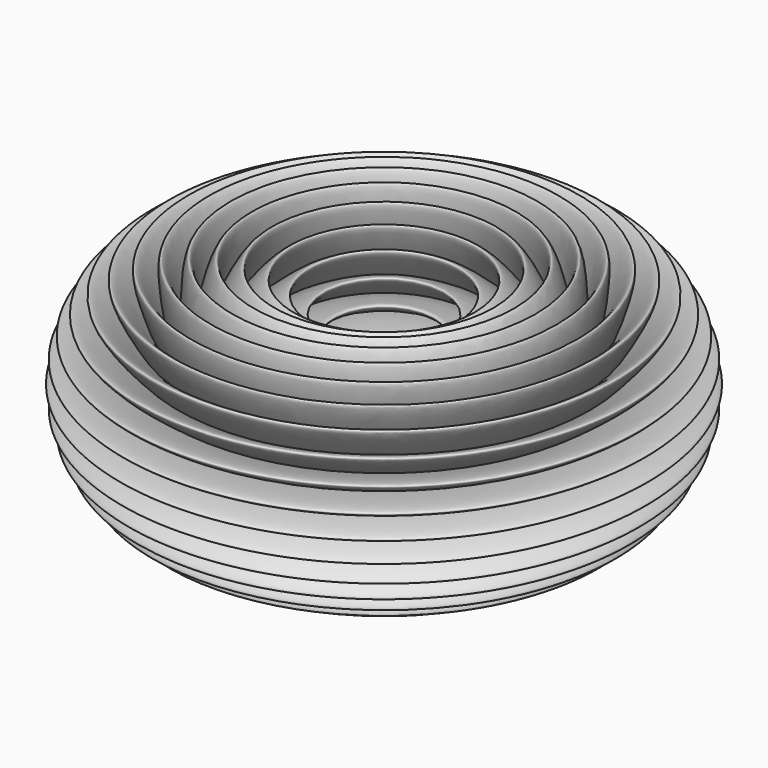
from build123d import *


with BuildPart() as f1:
    # F0 (on Front) → F1 (revolve)
    with BuildSketch(Plane.XZ):
        with BuildLine():
            add(Edge.make_bspline(
                [(306.7410461047, -30.2113560981), (430.4049725454, -21.4052719132), (586.5438764123, 0)],
                knots=[0.7817357195, 0.7817357195, 0.7817357195, 1.1221060483, 1.1221060483, 1.1221060483], degree=2, weights=[1, 0.9855534235, 1]))
            add(Edge.make_bspline(
                [(575.2736002958, -114.4290337258), (426.3108230752, -62.9738690757), (306.7410461047, -30.2113560981)],
                knots=[5.1610792589, 5.1610792589, 5.1610792589, 5.5014495877, 5.5014495877, 5.5014495877], degree=2, weights=[1, 0.9855534235, 1]))
            add(Edge.make_bspline(
                [(575.2736002958, -114.4290337259), (901.5747774696, -134.0658692103), (1253.6743252134, -123.4761436431)],
                knots=[1.1221060483, 1.1221060483, 1.1221060483, 1.8069156759, 1.8069156759, 1.8069156759], degree=2, weights=[1, 0.9419499659, 1]))
            add(Edge.make_bspline(
                [(1253.6743252134, -123.4761436431), (910.4062245206, -44.3986825322), (586.5438764123, 0)],
                knots=[4.4762696313, 4.4762696313, 4.4762696313, 5.1610792589, 5.1610792589, 5.1610792589], degree=2, weights=[1, 0.9419499659, 1]))
        make_face()
        with BuildLine():
            add(Edge.make_bspline(
                [(306.7410461047, 30.2113560981), (426.3108230753, 62.9738690757), (575.2736002958, 114.4290337258)],
                knots=[0.7817357195, 0.7817357195, 0.7817357195, 1.1221060483, 1.1221060483, 1.1221060483], degree=2, weights=[1, 0.9855534235, 1]))
            add(Edge.make_bspline(
                [(586.5438764123, 0), (430.4049725454, 21.4052719132), (306.7410461047, 30.2113560981)],
                knots=[5.1610792589, 5.1610792589, 5.1610792589, 5.5014495877, 5.5014495877, 5.5014495877], degree=2, weights=[1, 0.9855534235, 1]))
            add(Edge.make_bspline(
                [(586.5438764123, 0), (910.4062245206, 44.3986825322), (1253.6743252134, 123.4761436431)],
                knots=[1.1221060483, 1.1221060483, 1.1221060483, 1.8069156759, 1.8069156759, 1.8069156759], degree=2, weights=[1, 0.9419499659, 1]))
            add(Edge.make_bspline(
                [(1253.6743252134, 123.4761436431), (901.5747774696, 134.0658692103), (575.2736002958, 114.4290337259)],
                knots=[4.4762696313, 4.4762696313, 4.4762696313, 5.1610792589, 5.1610792589, 5.1610792589], degree=2, weights=[1, 0.9419499659, 1]))
        make_face()
        with BuildLine():
            add(Edge.make_bspline(
                [(294.9531597252, 89.4730628222), (405.8337877522, 144.9329595922), (541.8958823372, 224.4606238582)],
                knots=[0.7817357195, 0.7817357195, 0.7817357195, 1.1221060483, 1.1221060483, 1.1221060483], degree=2, weights=[1, 0.9855534235, 1]))
            add(Edge.make_bspline(
                [(575.2736002958, 114.4290337259), (417.9589002944, 104.9618203067), (294.9531597252, 89.4730628222)],
                knots=[5.1610792589, 5.1610792589, 5.1610792589, 5.5014495877, 5.5014495877, 5.5014495877], degree=2, weights=[1, 0.9855534235, 1]))
            add(Edge.make_bspline(
                [(575.2736002958, 114.4290337258), (884.251270925, 221.1570178041), (1205.4963239641, 365.6833119754)],
                knots=[1.1221060483, 1.1221060483, 1.1221060483, 1.8069156759, 1.8069156759, 1.8069156759], degree=2, weights=[1, 0.9419499659, 1]))
            add(Edge.make_bspline(
                [(1205.4963239641, 365.6833119754), (858.0963173294, 307.3783447841), (541.8958823372, 224.4606238582)],
                knots=[4.4762696313, 4.4762696313, 4.4762696313, 5.1610792589, 5.1610792589, 5.1610792589], degree=2, weights=[1, 0.9419499659, 1]))
        make_face()
        with BuildLine():
            add(Edge.make_bspline(
                [(575.2736002958, -114.4290337259), (901.5747774696, -134.0658692103), (1253.6743252134, -123.4761436431)],
                knots=[1.1221060483, 1.1221060483, 1.1221060483, 1.8069156759, 1.8069156759, 1.8069156759], degree=2, weights=[1, 0.9419499659, 1]))
            add(Edge.make_bspline(
                [(1205.4963239641, -365.6833119754), (884.251270925, -221.1570178041), (575.2736002958, -114.4290337258)],
                knots=[4.4762696313, 4.4762696313, 4.4762696313, 5.1610792589, 5.1610792589, 5.1610792589], degree=2, weights=[1, 0.9419499659, 1]))
            add(Edge.make_bspline(
                [(1205.4963239641, -365.6833119754), (1973.4335346691, -494.5680356943), (1992.9556897794, -396.4235343368), (2012.4778448897, -298.2790329793), (1253.6743252134, -123.4761436431)],
                knots=[1.8069156759, 1.8069156759, 1.8069156759, 3.1415926536, 3.1415926536, 4.4762696313, 4.4762696313, 4.4762696313], degree=2, weights=[1, 0.7854716489, 1, 0.7854716489, 1]))
        make_face()
        with BuildLine():
            add(Edge.make_bspline(
                [(1205.4963239641, -365.6833119754), (884.251270925, -221.1570178041), (575.2736002958, -114.4290337258)],
                knots=[4.4762696313, 4.4762696313, 4.4762696313, 5.1610792589, 5.1610792589, 5.1610792589], degree=2, weights=[1, 0.9419499659, 1]))
            add(Edge.make_bspline(
                [(294.9531597252, -89.4730628222), (417.9589002944, -104.9618203067), (575.2736002958, -114.4290337259)],
                knots=[0.7817357195, 0.7817357195, 0.7817357195, 1.1221060483, 1.1221060483, 1.1221060483], degree=2, weights=[1, 0.9855534235, 1]))
            add(Edge.make_bspline(
                [(541.8958823372, -224.4606238582), (405.8337877522, -144.9329595922), (294.9531597252, -89.4730628221)],
                knots=[5.1610792589, 5.1610792589, 5.1610792589, 5.5014495877, 5.5014495877, 5.5014495877], degree=2, weights=[1, 0.9855534235, 1]))
            add(Edge.make_bspline(
                [(541.8958823372, -224.4606238582), (858.0963173294, -307.3783447841), (1205.4963239641, -365.6833119754)],
                knots=[1.1221060483, 1.1221060483, 1.1221060483, 1.8069156759, 1.8069156759, 1.8069156759], degree=2, weights=[1, 0.9419499659, 1]))
        make_face()
        with BuildLine():
            add(Edge.make_bspline(
                [(586.5438764123, 0), (910.4062245206, 44.3986825322), (1253.6743252134, 123.4761436431)],
                knots=[1.1221060483, 1.1221060483, 1.1221060483, 1.8069156759, 1.8069156759, 1.8069156759], degree=2, weights=[1, 0.9419499659, 1]))
            add(Edge.make_bspline(
                [(1253.6743252134, -123.4761436431), (910.4062245206, -44.3986825322), (586.5438764123, 0)],
                knots=[4.4762696313, 4.4762696313, 4.4762696313, 5.1610792589, 5.1610792589, 5.1610792589], degree=2, weights=[1, 0.9419499659, 1]))
            add(Edge.make_bspline(
                [(1253.6743252134, -123.4761436431), (2032, -100.0672658109), (2032, 0), (2032, 100.0672658109), (1253.6743252134, 123.4761436431)],
                knots=[1.8069156759, 1.8069156759, 1.8069156759, 3.1415926536, 3.1415926536, 4.4762696313, 4.4762696313, 4.4762696313], degree=2, weights=[1, 0.7854716489, 1, 0.7854716489, 1]))
        make_face()
        with BuildLine():
            add(Edge.make_bspline(
                [(575.2736002958, 114.4290337258), (884.251270925, 221.1570178041), (1205.4963239641, 365.6833119754)],
                knots=[1.1221060483, 1.1221060483, 1.1221060483, 1.8069156759, 1.8069156759, 1.8069156759], degree=2, weights=[1, 0.9419499659, 1]))
            add(Edge.make_bspline(
                [(1253.6743252134, 123.4761436431), (901.5747774696, 134.0658692103), (575.2736002958, 114.4290337259)],
                knots=[4.4762696313, 4.4762696313, 4.4762696313, 5.1610792589, 5.1610792589, 5.1610792589], degree=2, weights=[1, 0.9419499659, 1]))
            add(Edge.make_bspline(
                [(1253.6743252134, 123.4761436431), (2012.4778448897, 298.2790329793), (1992.9556897794, 396.4235343368), (1973.4335346691, 494.5680356943), (1205.4963239641, 365.6833119754)],
                knots=[1.8069156759, 1.8069156759, 1.8069156759, 3.1415926536, 3.1415926536, 4.4762696313, 4.4762696313, 4.4762696313], degree=2, weights=[1, 0.7854716489, 1, 0.7854716489, 1]))
        make_face()
        with BuildLine():
            add(Edge.make_bspline(
                [(541.8958823372, 224.4606238582), (824.1150368816, 389.4164129081), (1110.991775035, 593.837475706)],
                knots=[1.1221060483, 1.1221060483, 1.1221060483, 1.8069156759, 1.8069156759, 1.8069156759], degree=2, weights=[1, 0.9419499659, 1]))
            add(Edge.make_bspline(
                [(1205.4963239641, 365.6833119754), (858.0963173294, 307.3783447841), (541.8958823372, 224.4606238582)],
                knots=[4.4762696313, 4.4762696313, 4.4762696313, 5.1610792589, 5.1610792589, 5.1610792589], degree=2, weights=[1, 0.9419499659, 1]))
            add(Edge.make_bspline(
                [(1205.4963239641, 365.6833119754), (1915.6172948108, 685.1626358088), (1877.3232100629, 777.6127345659), (1839.029125315, 870.0628333229), (1110.991775035, 593.837475706)],
                knots=[1.8069156759, 1.8069156759, 1.8069156759, 3.1415926536, 3.1415926536, 4.4762696313, 4.4762696313, 4.4762696313], degree=2, weights=[1, 0.7854716489, 1, 0.7854716489, 1]))
        make_face()
        with BuildLine():
            add(Edge.make_bspline(
                [(541.8958823372, 224.4606238582), (389.4509018993, 184.4847448091), (271.8303888292, 145.296369919)],
                knots=[5.1610792589, 5.1610792589, 5.1610792589, 5.5014495877, 5.5014495877, 5.5014495877], degree=2, weights=[1, 0.9855534235, 1]))
            add(Edge.make_bspline(
                [(541.8958823372, 224.4606238582), (824.1150368816, 389.4164129081), (1110.991775035, 593.837475706)],
                knots=[1.1221060483, 1.1221060483, 1.1221060483, 1.8069156759, 1.8069156759, 1.8069156759], degree=2, weights=[1, 0.9419499659, 1]))
            add(Edge.make_bspline(
                [(1110.991775035, 593.837475706), (781.6416969402, 468.8784429476), (487.6934095189, 325.8663180946)],
                knots=[4.4762696313, 4.4762696313, 4.4762696313, 5.1610792589, 5.1610792589, 5.1610792589], degree=2, weights=[1, 0.9419499659, 1]))
            add(Edge.make_bspline(
                [(271.8303888292, 145.296369919), (369.7607875601, 221.3223577509), (487.6934095189, 325.8663180946)],
                knots=[0.7817357195, 0.7817357195, 0.7817357195, 1.1221060483, 1.1221060483, 1.1221060483], degree=2, weights=[1, 0.9855534235, 1]))
        make_face()
        with BuildLine():
            add(Edge.make_bspline(
                [(1110.991775035, -593.8374757059), (1839.029125315, -870.0628333229), (1877.3232100629, -777.6127345659), (1915.6172948108, -685.1626358088), (1205.4963239641, -365.6833119754)],
                knots=[1.8069156759, 1.8069156759, 1.8069156759, 3.1415926536, 3.1415926536, 4.4762696313, 4.4762696313, 4.4762696313], degree=2, weights=[1, 0.7854716489, 1, 0.7854716489, 1]))
            add(Edge.make_bspline(
                [(541.8958823372, -224.4606238582), (858.0963173294, -307.3783447841), (1205.4963239641, -365.6833119754)],
                knots=[1.1221060483, 1.1221060483, 1.1221060483, 1.8069156759, 1.8069156759, 1.8069156759], degree=2, weights=[1, 0.9419499659, 1]))
            add(Edge.make_bspline(
                [(1110.991775035, -593.8374757059), (824.1150368816, -389.4164129081), (541.8958823372, -224.4606238582)],
                knots=[4.4762696313, 4.4762696313, 4.4762696313, 5.1610792589, 5.1610792589, 5.1610792589], degree=2, weights=[1, 0.9419499659, 1]))
        make_face()
        with BuildLine():
            add(Edge.make_bspline(
                [(1110.991775035, -593.8374757059), (824.1150368816, -389.4164129081), (541.8958823372, -224.4606238582)],
                knots=[4.4762696313, 4.4762696313, 4.4762696313, 5.1610792589, 5.1610792589, 5.1610792589], degree=2, weights=[1, 0.9419499659, 1]))
            add(Edge.make_bspline(
                [(271.8303888292, -145.296369919), (389.4509018993, -184.4847448091), (541.8958823372, -224.4606238582)],
                knots=[0.7817357195, 0.7817357195, 0.7817357195, 1.1221060483, 1.1221060483, 1.1221060483], degree=2, weights=[1, 0.9855534235, 1]))
            add(Edge.make_bspline(
                [(487.6934095189, -325.8663180946), (369.76078756, -221.3223577509), (271.8303888292, -145.296369919)],
                knots=[5.1610792589, 5.1610792589, 5.1610792589, 5.5014495877, 5.5014495877, 5.5014495877], degree=2, weights=[1, 0.9855534235, 1]))
            add(Edge.make_bspline(
                [(487.6934095189, -325.8663180946), (781.6416969401, -468.8784429476), (1110.991775035, -593.8374757059)],
                knots=[1.1221060483, 1.1221060483, 1.1221060483, 1.8069156759, 1.8069156759, 1.8069156759], degree=2, weights=[1, 0.9419499659, 1]))
        make_face()
        with BuildLine():
            add(Edge.make_bspline(
                [(1110.991775035, 593.837475706), (781.6416969402, 468.8784429476), (487.6934095189, 325.8663180946)],
                knots=[4.4762696313, 4.4762696313, 4.4762696313, 5.1610792589, 5.1610792589, 5.1610792589], degree=2, weights=[1, 0.9419499659, 1]))
            add(Edge.make_bspline(
                [(1110.991775035, 593.837475706), (1745.140646383, 1045.7158227879), (1689.5462521988, 1128.9187134958), (1633.9518580146, 1212.1216042038), (973.7924352426, 799.170798273)],
                knots=[1.8069156759, 1.8069156759, 1.8069156759, 3.1415926536, 3.1415926536, 4.4762696313, 4.4762696313, 4.4762696313], degree=2, weights=[1, 0.7854716489, 1, 0.7854716489, 1]))
            add(Edge.make_bspline(
                [(487.6934095189, 325.8663180946), (732.3085241398, 542.7107536512), (973.7924352426, 799.170798273)],
                knots=[1.1221060483, 1.1221060483, 1.1221060483, 1.8069156759, 1.8069156759, 1.8069156759], degree=2, weights=[1, 0.9419499659, 1]))
        make_face()
        with BuildLine():
            add(Edge.make_bspline(
                [(973.7924352426, -799.170798273), (1633.9518580146, -1212.1216042038), (1689.5462521988, -1128.9187134958), (1745.140646383, -1045.7158227879), (1110.991775035, -593.8374757059)],
                knots=[1.8069156759, 1.8069156759, 1.8069156759, 3.1415926536, 3.1415926536, 4.4762696313, 4.4762696313, 4.4762696313], degree=2, weights=[1, 0.7854716489, 1, 0.7854716489, 1]))
            add(Edge.make_bspline(
                [(487.6934095189, -325.8663180946), (781.6416969401, -468.8784429476), (1110.991775035, -593.8374757059)],
                knots=[1.1221060483, 1.1221060483, 1.1221060483, 1.8069156759, 1.8069156759, 1.8069156759], degree=2, weights=[1, 0.9419499659, 1]))
            add(Edge.make_bspline(
                [(973.7924352426, -799.170798273), (732.3085241398, -542.7107536512), (487.6934095189, -325.8663180946)],
                knots=[4.4762696313, 4.4762696313, 4.4762696313, 5.1610792589, 5.1610792589, 5.1610792589], degree=2, weights=[1, 0.9419499659, 1]))
        make_face()
        with BuildLine():
            add(Edge.make_bspline(
                [(487.6934095189, 325.8663180946), (345.9765237507, 256.9180240287), (238.2613285347, 195.5360190031)],
                knots=[5.1610792589, 5.1610792589, 5.1610792589, 5.5014495877, 5.5014495877, 5.5014495877], degree=2, weights=[1, 0.9855534235, 1]))
            add(Edge.make_bspline(
                [(487.6934095189, 325.8663180946), (732.3085241398, 542.7107536512), (973.7924352426, 799.170798273)],
                knots=[1.1221060483, 1.1221060483, 1.1221060483, 1.8069156759, 1.8069156759, 1.8069156759], degree=2, weights=[1, 0.9419499659, 1]))
            add(Edge.make_bspline(
                [(973.7924352426, 799.170798273), (675.1490244872, 612.3598054987), (414.7491524746, 414.7491524746)],
                knots=[4.4762696313, 4.4762696313, 4.4762696313, 5.1610792589, 5.1610792589, 5.1610792589], degree=2, weights=[1, 0.9419499659, 1]))
            add(Edge.make_bspline(
                [(238.2613285347, 195.5360190031), (319.4780876662, 289.2064618203), (414.7491524746, 414.7491524746)],
                knots=[0.7817357195, 0.7817357195, 0.7817357195, 1.1221060483, 1.1221060483, 1.1221060483], degree=2, weights=[1, 0.9855534235, 1]))
        make_face()
        with BuildLine():
            add(Edge.make_bspline(
                [(973.7924352426, 799.170798273), (675.1490244872, 612.3598054987), (414.7491524746, 414.7491524746)],
                knots=[4.4762696313, 4.4762696313, 4.4762696313, 5.1610792589, 5.1610792589, 5.1610792589], degree=2, weights=[1, 0.9419499659, 1]))
            add(Edge.make_bspline(
                [(973.7924352426, 799.170798273), (1507.5992216007, 1366.0827371414), (1436.8409793711, 1436.8409793711), (1366.0827371414, 1507.5992216007), (799.170798273, 973.7924352426)],
                knots=[1.8069156759, 1.8069156759, 1.8069156759, 3.1415926536, 3.1415926536, 4.4762696313, 4.4762696313, 4.4762696313], degree=2, weights=[1, 0.7854716489, 1, 0.7854716489, 1]))
            add(Edge.make_bspline(
                [(414.7491524746, 414.7491524746), (612.3598054987, 675.1490244872), (799.170798273, 973.7924352426)],
                knots=[1.1221060483, 1.1221060483, 1.1221060483, 1.8069156759, 1.8069156759, 1.8069156759], degree=2, weights=[1, 0.9419499659, 1]))
        make_face()
        with BuildLine():
            add(Edge.make_bspline(
                [(414.7491524746, -414.7491524746), (675.1490244872, -612.3598054987), (973.7924352426, -799.170798273)],
                knots=[1.1221060483, 1.1221060483, 1.1221060483, 1.8069156759, 1.8069156759, 1.8069156759], degree=2, weights=[1, 0.9419499659, 1]))
            add(Edge.make_bspline(
                [(973.7924352426, -799.170798273), (732.3085241398, -542.7107536512), (487.6934095189, -325.8663180946)],
                knots=[4.4762696313, 4.4762696313, 4.4762696313, 5.1610792589, 5.1610792589, 5.1610792589], degree=2, weights=[1, 0.9419499659, 1]))
            add(Edge.make_bspline(
                [(238.2613285347, -195.5360190031), (345.9765237507, -256.9180240287), (487.6934095189, -325.8663180946)],
                knots=[0.7817357195, 0.7817357195, 0.7817357195, 1.1221060483, 1.1221060483, 1.1221060483], degree=2, weights=[1, 0.9855534235, 1]))
            add(Edge.make_bspline(
                [(414.7491524746, -414.7491524746), (319.4780876662, -289.2064618203), (238.2613285347, -195.5360190031)],
                knots=[5.1610792589, 5.1610792589, 5.1610792589, 5.5014495877, 5.5014495877, 5.5014495877], degree=2, weights=[1, 0.9855534235, 1]))
        make_face()
        with BuildLine():
            add(Edge.make_bspline(
                [(799.170798273, -973.7924352426), (1366.0827371414, -1507.5992216008), (1436.8409793711, -1436.8409793711), (1507.5992216007, -1366.0827371414), (973.7924352426, -799.170798273)],
                knots=[1.8069156759, 1.8069156759, 1.8069156759, 3.1415926536, 3.1415926536, 4.4762696313, 4.4762696313, 4.4762696313], degree=2, weights=[1, 0.7854716489, 1, 0.7854716489, 1]))
            add(Edge.make_bspline(
                [(414.7491524746, -414.7491524746), (675.1490244872, -612.3598054987), (973.7924352426, -799.170798273)],
                knots=[1.1221060483, 1.1221060483, 1.1221060483, 1.8069156759, 1.8069156759, 1.8069156759], degree=2, weights=[1, 0.9419499659, 1]))
            add(Edge.make_bspline(
                [(799.170798273, -973.7924352426), (612.3598054987, -675.1490244873), (414.7491524746, -414.7491524746)],
                knots=[4.4762696313, 4.4762696313, 4.4762696313, 5.1610792589, 5.1610792589, 5.1610792589], degree=2, weights=[1, 0.9419499659, 1]))
        make_face()
        with BuildLine():
            add(Edge.make_bspline(
                [(414.7491524746, 414.7491524746), (289.2064618203, 319.4780876662), (195.5360190031, 238.2613285347)],
                knots=[5.1610792589, 5.1610792589, 5.1610792589, 5.5014495877, 5.5014495877, 5.5014495877], degree=2, weights=[1, 0.9855534235, 1]))
            add(Edge.make_bspline(
                [(414.7491524746, 414.7491524746), (612.3598054987, 675.1490244872), (799.170798273, 973.7924352426)],
                knots=[1.1221060483, 1.1221060483, 1.1221060483, 1.8069156759, 1.8069156759, 1.8069156759], degree=2, weights=[1, 0.9419499659, 1]))
            add(Edge.make_bspline(
                [(799.170798273, 973.7924352426), (542.7107536512, 732.3085241398), (325.8663180946, 487.6934095189)],
                knots=[4.4762696313, 4.4762696313, 4.4762696313, 5.1610792589, 5.1610792589, 5.1610792589], degree=2, weights=[1, 0.9419499659, 1]))
            add(Edge.make_bspline(
                [(195.5360190031, 238.2613285347), (256.9180240287, 345.9765237507), (325.8663180946, 487.6934095189)],
                knots=[0.7817357195, 0.7817357195, 0.7817357195, 1.1221060483, 1.1221060483, 1.1221060483], degree=2, weights=[1, 0.9855534235, 1]))
        make_face()
        with BuildLine():
            add(Edge.make_bspline(
                [(799.170798273, 973.7924352426), (542.7107536512, 732.3085241398), (325.8663180946, 487.6934095189)],
                knots=[4.4762696313, 4.4762696313, 4.4762696313, 5.1610792589, 5.1610792589, 5.1610792589], degree=2, weights=[1, 0.9419499659, 1]))
            add(Edge.make_bspline(
                [(799.170798273, 973.7924352426), (1212.1216042038, 1633.9518580145), (1128.9187134958, 1689.5462521988), (1045.7158227879, 1745.140646383), (593.837475706, 1110.991775035)],
                knots=[1.8069156759, 1.8069156759, 1.8069156759, 3.1415926536, 3.1415926536, 4.4762696313, 4.4762696313, 4.4762696313], degree=2, weights=[1, 0.7854716489, 1, 0.7854716489, 1]))
            add(Edge.make_bspline(
                [(325.8663180946, 487.6934095189), (468.8784429476, 781.6416969402), (593.837475706, 1110.9917750351)],
                knots=[1.1221060483, 1.1221060483, 1.1221060483, 1.8069156759, 1.8069156759, 1.8069156759], degree=2, weights=[1, 0.9419499659, 1]))
        make_face()
        with BuildLine():
            add(Edge.make_bspline(
                [(325.8663180946, -487.6934095189), (542.7107536512, -732.3085241398), (799.170798273, -973.7924352426)],
                knots=[1.1221060483, 1.1221060483, 1.1221060483, 1.8069156759, 1.8069156759, 1.8069156759], degree=2, weights=[1, 0.9419499659, 1]))
            add(Edge.make_bspline(
                [(799.170798273, -973.7924352426), (612.3598054987, -675.1490244873), (414.7491524746, -414.7491524746)],
                knots=[4.4762696313, 4.4762696313, 4.4762696313, 5.1610792589, 5.1610792589, 5.1610792589], degree=2, weights=[1, 0.9419499659, 1]))
            add(Edge.make_bspline(
                [(195.5360190031, -238.2613285347), (289.2064618203, -319.4780876662), (414.7491524746, -414.7491524746)],
                knots=[0.7817357195, 0.7817357195, 0.7817357195, 1.1221060483, 1.1221060483, 1.1221060483], degree=2, weights=[1, 0.9855534235, 1]))
            add(Edge.make_bspline(
                [(325.8663180946, -487.6934095189), (256.9180240287, -345.9765237507), (195.5360190031, -238.2613285347)],
                knots=[5.1610792589, 5.1610792589, 5.1610792589, 5.5014495877, 5.5014495877, 5.5014495877], degree=2, weights=[1, 0.9855534235, 1]))
        make_face()
        with BuildLine():
            add(Edge.make_bspline(
                [(593.8374757059, -1110.991775035), (1045.7158227879, -1745.140646383), (1128.9187134958, -1689.5462521988), (1212.1216042038, -1633.9518580146), (799.170798273, -973.7924352426)],
                knots=[1.8069156759, 1.8069156759, 1.8069156759, 3.1415926536, 3.1415926536, 4.4762696313, 4.4762696313, 4.4762696313], degree=2, weights=[1, 0.7854716489, 1, 0.7854716489, 1]))
            add(Edge.make_bspline(
                [(325.8663180946, -487.6934095189), (542.7107536512, -732.3085241398), (799.170798273, -973.7924352426)],
                knots=[1.1221060483, 1.1221060483, 1.1221060483, 1.8069156759, 1.8069156759, 1.8069156759], degree=2, weights=[1, 0.9419499659, 1]))
            add(Edge.make_bspline(
                [(593.8374757059, -1110.991775035), (468.8784429476, -781.6416969402), (325.8663180946, -487.6934095189)],
                knots=[4.4762696313, 4.4762696313, 4.4762696313, 5.1610792589, 5.1610792589, 5.1610792589], degree=2, weights=[1, 0.9419499659, 1]))
        make_face()
        with BuildLine():
            add(Edge.make_bspline(
                [(593.837475706, 1110.991775035), (389.4164129081, 824.1150368816), (224.4606238582, 541.8958823372)],
                knots=[4.4762696313, 4.4762696313, 4.4762696313, 5.1610792589, 5.1610792589, 5.1610792589], degree=2, weights=[1, 0.9419499659, 1]))
            add(Edge.make_bspline(
                [(593.837475706, 1110.9917750351), (870.0628333229, 1839.0291253151), (777.6127345659, 1877.3232100629), (685.1626358088, 1915.6172948108), (365.6833119754, 1205.4963239641)],
                knots=[1.8069156759, 1.8069156759, 1.8069156759, 3.1415926536, 3.1415926536, 4.4762696313, 4.4762696313, 4.4762696313], degree=2, weights=[1, 0.7854716489, 1, 0.7854716489, 1]))
            add(Edge.make_bspline(
                [(224.4606238582, 541.8958823372), (307.3783447841, 858.0963173294), (365.6833119754, 1205.4963239641)],
                knots=[1.1221060483, 1.1221060483, 1.1221060483, 1.8069156759, 1.8069156759, 1.8069156759], degree=2, weights=[1, 0.9419499659, 1]))
        make_face()
        with BuildLine():
            add(Edge.make_bspline(
                [(325.8663180946, 487.6934095189), (468.8784429476, 781.6416969402), (593.837475706, 1110.9917750351)],
                knots=[1.1221060483, 1.1221060483, 1.1221060483, 1.8069156759, 1.8069156759, 1.8069156759], degree=2, weights=[1, 0.9419499659, 1]))
            add(Edge.make_bspline(
                [(593.837475706, 1110.991775035), (389.4164129081, 824.1150368816), (224.4606238582, 541.8958823372)],
                knots=[4.4762696313, 4.4762696313, 4.4762696313, 5.1610792589, 5.1610792589, 5.1610792589], degree=2, weights=[1, 0.9419499659, 1]))
            add(Edge.make_bspline(
                [(145.296369919, 271.8303888292), (184.4847448091, 389.4509018993), (224.4606238582, 541.8958823372)],
                knots=[0.7817357195, 0.7817357195, 0.7817357195, 1.1221060483, 1.1221060483, 1.1221060483], degree=2, weights=[1, 0.9855534235, 1]))
            add(Edge.make_bspline(
                [(325.8663180946, 487.6934095189), (221.3223577509, 369.7607875601), (145.296369919, 271.8303888292)],
                knots=[5.1610792589, 5.1610792589, 5.1610792589, 5.5014495877, 5.5014495877, 5.5014495877], degree=2, weights=[1, 0.9855534235, 1]))
        make_face()
        with BuildLine():
            add(Edge.make_bspline(
                [(365.6833119753, -1205.4963239641), (685.1626358088, -1915.6172948108), (777.6127345659, -1877.3232100629), (870.0628333229, -1839.029125315), (593.8374757059, -1110.991775035)],
                knots=[1.8069156759, 1.8069156759, 1.8069156759, 3.1415926536, 3.1415926536, 4.4762696313, 4.4762696313, 4.4762696313], degree=2, weights=[1, 0.7854716489, 1, 0.7854716489, 1]))
            add(Edge.make_bspline(
                [(224.4606238582, -541.8958823372), (389.4164129081, -824.1150368816), (593.8374757059, -1110.991775035)],
                knots=[1.1221060483, 1.1221060483, 1.1221060483, 1.8069156759, 1.8069156759, 1.8069156759], degree=2, weights=[1, 0.9419499659, 1]))
            add(Edge.make_bspline(
                [(365.6833119753, -1205.4963239641), (307.3783447841, -858.0963173294), (224.4606238582, -541.8958823372)],
                knots=[4.4762696313, 4.4762696313, 4.4762696313, 5.1610792589, 5.1610792589, 5.1610792589], degree=2, weights=[1, 0.9419499659, 1]))
        make_face()
        with BuildLine():
            add(Edge.make_bspline(
                [(224.4606238582, -541.8958823372), (389.4164129081, -824.1150368816), (593.8374757059, -1110.991775035)],
                knots=[1.1221060483, 1.1221060483, 1.1221060483, 1.8069156759, 1.8069156759, 1.8069156759], degree=2, weights=[1, 0.9419499659, 1]))
            add(Edge.make_bspline(
                [(593.8374757059, -1110.991775035), (468.8784429476, -781.6416969402), (325.8663180946, -487.6934095189)],
                knots=[4.4762696313, 4.4762696313, 4.4762696313, 5.1610792589, 5.1610792589, 5.1610792589], degree=2, weights=[1, 0.9419499659, 1]))
            add(Edge.make_bspline(
                [(145.296369919, -271.8303888292), (221.3223577509, -369.7607875601), (325.8663180946, -487.6934095189)],
                knots=[0.7817357195, 0.7817357195, 0.7817357195, 1.1221060483, 1.1221060483, 1.1221060483], degree=2, weights=[1, 0.9855534235, 1]))
            add(Edge.make_bspline(
                [(224.4606238582, -541.8958823372), (184.4847448091, -389.4509018993), (145.296369919, -271.8303888292)],
                knots=[5.1610792589, 5.1610792589, 5.1610792589, 5.5014495877, 5.5014495877, 5.5014495877], degree=2, weights=[1, 0.9855534235, 1]))
        make_face()
        with BuildLine():
            add(Edge.make_bspline(
                [(365.6833119754, 1205.4963239641), (221.1570178041, 884.251270925), (114.4290337258, 575.2736002958)],
                knots=[4.4762696313, 4.4762696313, 4.4762696313, 5.1610792589, 5.1610792589, 5.1610792589], degree=2, weights=[1, 0.9419499659, 1]))
            add(Edge.make_bspline(
                [(365.6833119754, 1205.4963239641), (494.5680356943, 1973.4335346691), (396.4235343368, 1992.9556897794), (298.2790329793, 2012.4778448897), (123.4761436431, 1253.6743252134)],
                knots=[1.8069156759, 1.8069156759, 1.8069156759, 3.1415926536, 3.1415926536, 4.4762696313, 4.4762696313, 4.4762696313], degree=2, weights=[1, 0.7854716489, 1, 0.7854716489, 1]))
            add(Edge.make_bspline(
                [(114.4290337259, 575.2736002958), (134.0658692103, 901.5747774696), (123.4761436431, 1253.6743252134)],
                knots=[1.1221060483, 1.1221060483, 1.1221060483, 1.8069156759, 1.8069156759, 1.8069156759], degree=2, weights=[1, 0.9419499659, 1]))
        make_face()
        with BuildLine():
            add(Edge.make_bspline(
                [(224.4606238582, 541.8958823372), (307.3783447841, 858.0963173294), (365.6833119754, 1205.4963239641)],
                knots=[1.1221060483, 1.1221060483, 1.1221060483, 1.8069156759, 1.8069156759, 1.8069156759], degree=2, weights=[1, 0.9419499659, 1]))
            add(Edge.make_bspline(
                [(365.6833119754, 1205.4963239641), (221.1570178041, 884.251270925), (114.4290337258, 575.2736002958)],
                knots=[4.4762696313, 4.4762696313, 4.4762696313, 5.1610792589, 5.1610792589, 5.1610792589], degree=2, weights=[1, 0.9419499659, 1]))
            add(Edge.make_bspline(
                [(89.4730628222, 294.9531597252), (104.9618203067, 417.9589002944), (114.4290337259, 575.2736002958)],
                knots=[0.7817357195, 0.7817357195, 0.7817357195, 1.1221060483, 1.1221060483, 1.1221060483], degree=2, weights=[1, 0.9855534235, 1]))
            add(Edge.make_bspline(
                [(224.4606238582, 541.8958823372), (144.9329595922, 405.8337877522), (89.4730628222, 294.9531597252)],
                knots=[5.1610792589, 5.1610792589, 5.1610792589, 5.5014495877, 5.5014495877, 5.5014495877], degree=2, weights=[1, 0.9855534235, 1]))
        make_face()
        with BuildLine():
            add(Edge.make_bspline(
                [(365.6833119753, -1205.4963239641), (307.3783447841, -858.0963173294), (224.4606238582, -541.8958823372)],
                knots=[4.4762696313, 4.4762696313, 4.4762696313, 5.1610792589, 5.1610792589, 5.1610792589], degree=2, weights=[1, 0.9419499659, 1]))
            add(Edge.make_bspline(
                [(89.4730628221, -294.9531597252), (144.9329595922, -405.8337877522), (224.4606238582, -541.8958823372)],
                knots=[0.7817357195, 0.7817357195, 0.7817357195, 1.1221060483, 1.1221060483, 1.1221060483], degree=2, weights=[1, 0.9855534235, 1]))
            add(Edge.make_bspline(
                [(114.4290337259, -575.2736002958), (104.9618203067, -417.9589002944), (89.4730628222, -294.9531597252)],
                knots=[5.1610792589, 5.1610792589, 5.1610792589, 5.5014495877, 5.5014495877, 5.5014495877], degree=2, weights=[1, 0.9855534235, 1]))
            add(Edge.make_bspline(
                [(114.4290337258, -575.2736002958), (221.1570178041, -884.251270925), (365.6833119753, -1205.4963239641)],
                knots=[1.1221060483, 1.1221060483, 1.1221060483, 1.8069156759, 1.8069156759, 1.8069156759], degree=2, weights=[1, 0.9419499659, 1]))
        make_face()
        with BuildLine():
            add(Edge.make_bspline(
                [(123.4761436431, -1253.6743252134), (298.2790329793, -2012.4778448897), (396.4235343368, -1992.9556897794), (494.5680356943, -1973.433534669), (365.6833119753, -1205.4963239641)],
                knots=[1.8069156759, 1.8069156759, 1.8069156759, 3.1415926536, 3.1415926536, 4.4762696313, 4.4762696313, 4.4762696313], degree=2, weights=[1, 0.7854716489, 1, 0.7854716489, 1]))
            add(Edge.make_bspline(
                [(114.4290337258, -575.2736002958), (221.1570178041, -884.251270925), (365.6833119753, -1205.4963239641)],
                knots=[1.1221060483, 1.1221060483, 1.1221060483, 1.8069156759, 1.8069156759, 1.8069156759], degree=2, weights=[1, 0.9419499659, 1]))
            add(Edge.make_bspline(
                [(123.4761436431, -1253.6743252134), (134.0658692103, -901.5747774696), (114.4290337259, -575.2736002958)],
                knots=[4.4762696313, 4.4762696313, 4.4762696313, 5.1610792589, 5.1610792589, 5.1610792589], degree=2, weights=[1, 0.9419499659, 1]))
        make_face()
        with BuildLine():
            add(Edge.make_bspline(
                [(123.4761436431, 1253.6743252134), (44.3986825322, 910.4062245206), (0, 586.5438764123)],
                knots=[4.4762696313, 4.4762696313, 4.4762696313, 5.1610792589, 5.1610792589, 5.1610792589], degree=2, weights=[1, 0.9419499659, 1]))
            add(Edge.make_bspline(
                [(123.4761436431, 1253.6743252134), (100.0672658109, 2032), (0, 2032), (-100.0672658109, 2032), (-123.4761436431, 1253.6743252133)],
                knots=[1.8069156759, 1.8069156759, 1.8069156759, 3.1415926536, 3.1415926536, 4.4762696313, 4.4762696313, 4.4762696313], degree=2, weights=[1, 0.7854716489, 1, 0.7854716489, 1]))
            add(Edge.make_bspline(
                [(0, 586.5438764123), (-44.3986825322, 910.4062245206), (-123.4761436431, 1253.6743252134)],
                knots=[1.1221060483, 1.1221060483, 1.1221060483, 1.8069156759, 1.8069156759, 1.8069156759], degree=2, weights=[1, 0.9419499659, 1]))
        make_face()
        with BuildLine():
            add(Edge.make_bspline(
                [(114.4290337259, 575.2736002958), (134.0658692103, 901.5747774696), (123.4761436431, 1253.6743252134)],
                knots=[1.1221060483, 1.1221060483, 1.1221060483, 1.8069156759, 1.8069156759, 1.8069156759], degree=2, weights=[1, 0.9419499659, 1]))
            add(Edge.make_bspline(
                [(123.4761436431, 1253.6743252134), (44.3986825322, 910.4062245206), (0, 586.5438764123)],
                knots=[4.4762696313, 4.4762696313, 4.4762696313, 5.1610792589, 5.1610792589, 5.1610792589], degree=2, weights=[1, 0.9419499659, 1]))
            add(Edge.make_bspline(
                [(30.2113560981, 306.7410461047), (21.4052719132, 430.4049725454), (0, 586.5438764123)],
                knots=[0.7817357195, 0.7817357195, 0.7817357195, 1.1221060483, 1.1221060483, 1.1221060483], degree=2, weights=[1, 0.9855534235, 1]))
            add(Edge.make_bspline(
                [(114.4290337258, 575.2736002958), (62.9738690757, 426.3108230752), (30.2113560981, 306.7410461047)],
                knots=[5.1610792589, 5.1610792589, 5.1610792589, 5.5014495877, 5.5014495877, 5.5014495877], degree=2, weights=[1, 0.9855534235, 1]))
        make_face()
        with BuildLine():
            add(Edge.make_bspline(
                [(123.4761436431, -1253.6743252134), (134.0658692103, -901.5747774696), (114.4290337259, -575.2736002958)],
                knots=[4.4762696313, 4.4762696313, 4.4762696313, 5.1610792589, 5.1610792589, 5.1610792589], degree=2, weights=[1, 0.9419499659, 1]))
            add(Edge.make_bspline(
                [(30.2113560981, -306.7410461047), (62.9738690757, -426.3108230752), (114.4290337258, -575.2736002958)],
                knots=[0.7817357195, 0.7817357195, 0.7817357195, 1.1221060483, 1.1221060483, 1.1221060483], degree=2, weights=[1, 0.9855534235, 1]))
            add(Edge.make_bspline(
                [(0, -586.5438764123), (21.4052719132, -430.4049725454), (30.2113560981, -306.7410461047)],
                knots=[5.1610792589, 5.1610792589, 5.1610792589, 5.5014495877, 5.5014495877, 5.5014495877], degree=2, weights=[1, 0.9855534235, 1]))
            add(Edge.make_bspline(
                [(0, -586.5438764123), (44.3986825322, -910.4062245206), (123.4761436431, -1253.6743252134)],
                knots=[1.1221060483, 1.1221060483, 1.1221060483, 1.8069156759, 1.8069156759, 1.8069156759], degree=2, weights=[1, 0.9419499659, 1]))
        make_face()
        with BuildLine():
            add(Edge.make_bspline(
                [(-123.4761436431, -1253.6743252134), (-100.0672658109, -2032), (0, -2032), (100.0672658109, -2032), (123.4761436431, -1253.6743252134)],
                knots=[1.8069156759, 1.8069156759, 1.8069156759, 3.1415926536, 3.1415926536, 4.4762696313, 4.4762696313, 4.4762696313], degree=2, weights=[1, 0.7854716489, 1, 0.7854716489, 1]))
            add(Edge.make_bspline(
                [(0, -586.5438764123), (44.3986825322, -910.4062245206), (123.4761436431, -1253.6743252134)],
                knots=[1.1221060483, 1.1221060483, 1.1221060483, 1.8069156759, 1.8069156759, 1.8069156759], degree=2, weights=[1, 0.9419499659, 1]))
            add(Edge.make_bspline(
                [(-123.4761436431, -1253.6743252134), (-44.3986825322, -910.4062245206), (0, -586.5438764123)],
                knots=[4.4762696313, 4.4762696313, 4.4762696313, 5.1610792589, 5.1610792589, 5.1610792589], degree=2, weights=[1, 0.9419499659, 1]))
        make_face()
        with BuildLine():
            add(Edge.make_bspline(
                [(0, 586.5438764123), (-44.3986825322, 910.4062245206), (-123.4761436431, 1253.6743252134)],
                knots=[1.1221060483, 1.1221060483, 1.1221060483, 1.8069156759, 1.8069156759, 1.8069156759], degree=2, weights=[1, 0.9419499659, 1]))
            add(Edge.make_bspline(
                [(-123.4761436431, 1253.6743252133), (-134.0658692103, 901.5747774696), (-114.4290337259, 575.2736002958)],
                knots=[4.4762696313, 4.4762696313, 4.4762696313, 5.1610792589, 5.1610792589, 5.1610792589], degree=2, weights=[1, 0.9419499659, 1]))
            add(Edge.make_bspline(
                [(-30.2113560981, 306.7410461047), (-62.9738690757, 426.3108230752), (-114.4290337258, 575.2736002958)],
                knots=[0.7817357195, 0.7817357195, 0.7817357195, 1.1221060483, 1.1221060483, 1.1221060483], degree=2, weights=[1, 0.9855534235, 1]))
            add(Edge.make_bspline(
                [(0, 586.5438764123), (-21.4052719132, 430.4049725454), (-30.2113560981, 306.7410461047)],
                knots=[5.1610792589, 5.1610792589, 5.1610792589, 5.5014495877, 5.5014495877, 5.5014495877], degree=2, weights=[1, 0.9855534235, 1]))
        make_face()
        with BuildLine():
            add(Edge.make_bspline(
                [(-123.4761436431, 1253.6743252133), (-134.0658692103, 901.5747774696), (-114.4290337259, 575.2736002958)],
                knots=[4.4762696313, 4.4762696313, 4.4762696313, 5.1610792589, 5.1610792589, 5.1610792589], degree=2, weights=[1, 0.9419499659, 1]))
            add(Edge.make_bspline(
                [(-123.4761436431, 1253.6743252134), (-298.2790329793, 2012.4778448897), (-396.4235343368, 1992.9556897794), (-494.5680356943, 1973.4335346691), (-365.6833119754, 1205.4963239641)],
                knots=[1.8069156759, 1.8069156759, 1.8069156759, 3.1415926536, 3.1415926536, 4.4762696313, 4.4762696313, 4.4762696313], degree=2, weights=[1, 0.7854716489, 1, 0.7854716489, 1]))
            add(Edge.make_bspline(
                [(-114.4290337258, 575.2736002958), (-221.1570178041, 884.251270925), (-365.6833119754, 1205.4963239641)],
                knots=[1.1221060483, 1.1221060483, 1.1221060483, 1.8069156759, 1.8069156759, 1.8069156759], degree=2, weights=[1, 0.9419499659, 1]))
        make_face()
        with BuildLine():
            add(Edge.make_bspline(
                [(-123.4761436431, -1253.6743252134), (-44.3986825322, -910.4062245206), (0, -586.5438764123)],
                knots=[4.4762696313, 4.4762696313, 4.4762696313, 5.1610792589, 5.1610792589, 5.1610792589], degree=2, weights=[1, 0.9419499659, 1]))
            add(Edge.make_bspline(
                [(-30.2113560981, -306.7410461047), (-21.4052719132, -430.4049725454), (0, -586.5438764123)],
                knots=[0.7817357195, 0.7817357195, 0.7817357195, 1.1221060483, 1.1221060483, 1.1221060483], degree=2, weights=[1, 0.9855534235, 1]))
            add(Edge.make_bspline(
                [(-114.4290337258, -575.2736002958), (-62.9738690757, -426.3108230753), (-30.2113560981, -306.7410461047)],
                knots=[5.1610792589, 5.1610792589, 5.1610792589, 5.5014495877, 5.5014495877, 5.5014495877], degree=2, weights=[1, 0.9855534235, 1]))
            add(Edge.make_bspline(
                [(-114.4290337259, -575.2736002958), (-134.0658692103, -901.5747774696), (-123.4761436431, -1253.6743252134)],
                knots=[1.1221060483, 1.1221060483, 1.1221060483, 1.8069156759, 1.8069156759, 1.8069156759], degree=2, weights=[1, 0.9419499659, 1]))
        make_face()
        with BuildLine():
            add(Edge.make_bspline(
                [(-365.6833119754, -1205.4963239641), (-494.5680356943, -1973.433534669), (-396.4235343368, -1992.9556897794), (-298.2790329793, -2012.4778448897), (-123.4761436431, -1253.6743252134)],
                knots=[1.8069156759, 1.8069156759, 1.8069156759, 3.1415926536, 3.1415926536, 4.4762696313, 4.4762696313, 4.4762696313], degree=2, weights=[1, 0.7854716489, 1, 0.7854716489, 1]))
            add(Edge.make_bspline(
                [(-114.4290337259, -575.2736002958), (-134.0658692103, -901.5747774696), (-123.4761436431, -1253.6743252134)],
                knots=[1.1221060483, 1.1221060483, 1.1221060483, 1.8069156759, 1.8069156759, 1.8069156759], degree=2, weights=[1, 0.9419499659, 1]))
            add(Edge.make_bspline(
                [(-365.6833119754, -1205.4963239641), (-221.1570178041, -884.251270925), (-114.4290337258, -575.2736002958)],
                knots=[4.4762696313, 4.4762696313, 4.4762696313, 5.1610792589, 5.1610792589, 5.1610792589], degree=2, weights=[1, 0.9419499659, 1]))
        make_face()
        with BuildLine():
            add(Edge.make_bspline(
                [(-114.4290337259, 575.2736002958), (-104.9618203067, 417.9589002944), (-89.4730628222, 294.9531597252)],
                knots=[5.1610792589, 5.1610792589, 5.1610792589, 5.5014495877, 5.5014495877, 5.5014495877], degree=2, weights=[1, 0.9855534235, 1]))
            add(Edge.make_bspline(
                [(-114.4290337258, 575.2736002958), (-221.1570178041, 884.251270925), (-365.6833119754, 1205.4963239641)],
                knots=[1.1221060483, 1.1221060483, 1.1221060483, 1.8069156759, 1.8069156759, 1.8069156759], degree=2, weights=[1, 0.9419499659, 1]))
            add(Edge.make_bspline(
                [(-365.6833119754, 1205.4963239641), (-307.3783447841, 858.0963173294), (-224.4606238582, 541.8958823372)],
                knots=[4.4762696313, 4.4762696313, 4.4762696313, 5.1610792589, 5.1610792589, 5.1610792589], degree=2, weights=[1, 0.9419499659, 1]))
            add(Edge.make_bspline(
                [(-89.4730628221, 294.9531597252), (-144.9329595922, 405.8337877522), (-224.4606238582, 541.8958823372)],
                knots=[0.7817357195, 0.7817357195, 0.7817357195, 1.1221060483, 1.1221060483, 1.1221060483], degree=2, weights=[1, 0.9855534235, 1]))
        make_face()
        with BuildLine():
            add(Edge.make_bspline(
                [(-365.6833119754, 1205.4963239641), (-307.3783447841, 858.0963173294), (-224.4606238582, 541.8958823372)],
                knots=[4.4762696313, 4.4762696313, 4.4762696313, 5.1610792589, 5.1610792589, 5.1610792589], degree=2, weights=[1, 0.9419499659, 1]))
            add(Edge.make_bspline(
                [(-365.6833119754, 1205.4963239641), (-685.1626358088, 1915.6172948108), (-777.6127345659, 1877.3232100629), (-870.0628333229, 1839.029125315), (-593.8374757059, 1110.991775035)],
                knots=[1.8069156759, 1.8069156759, 1.8069156759, 3.1415926536, 3.1415926536, 4.4762696313, 4.4762696313, 4.4762696313], degree=2, weights=[1, 0.7854716489, 1, 0.7854716489, 1]))
            add(Edge.make_bspline(
                [(-224.4606238582, 541.8958823372), (-389.4164129081, 824.1150368816), (-593.8374757059, 1110.991775035)],
                knots=[1.1221060483, 1.1221060483, 1.1221060483, 1.8069156759, 1.8069156759, 1.8069156759], degree=2, weights=[1, 0.9419499659, 1]))
        make_face()
        with BuildLine():
            add(Edge.make_bspline(
                [(-224.4606238582, -541.8958823371), (-307.3783447841, -858.0963173294), (-365.6833119754, -1205.4963239641)],
                knots=[1.1221060483, 1.1221060483, 1.1221060483, 1.8069156759, 1.8069156759, 1.8069156759], degree=2, weights=[1, 0.9419499659, 1]))
            add(Edge.make_bspline(
                [(-365.6833119754, -1205.4963239641), (-221.1570178041, -884.251270925), (-114.4290337258, -575.2736002958)],
                knots=[4.4762696313, 4.4762696313, 4.4762696313, 5.1610792589, 5.1610792589, 5.1610792589], degree=2, weights=[1, 0.9419499659, 1]))
            add(Edge.make_bspline(
                [(-89.4730628222, -294.9531597252), (-104.9618203067, -417.9589002944), (-114.4290337259, -575.2736002958)],
                knots=[0.7817357195, 0.7817357195, 0.7817357195, 1.1221060483, 1.1221060483, 1.1221060483], degree=2, weights=[1, 0.9855534235, 1]))
            add(Edge.make_bspline(
                [(-224.4606238582, -541.8958823371), (-144.9329595922, -405.8337877522), (-89.4730628221, -294.9531597252)],
                knots=[5.1610792589, 5.1610792589, 5.1610792589, 5.5014495877, 5.5014495877, 5.5014495877], degree=2, weights=[1, 0.9855534235, 1]))
        make_face()
        with BuildLine():
            add(Edge.make_bspline(
                [(-593.8374757059, -1110.9917750349), (-870.0628333229, -1839.029125315), (-777.6127345659, -1877.3232100629), (-685.1626358088, -1915.6172948109), (-365.6833119754, -1205.4963239641)],
                knots=[1.8069156759, 1.8069156759, 1.8069156759, 3.1415926536, 3.1415926536, 4.4762696313, 4.4762696313, 4.4762696313], degree=2, weights=[1, 0.7854716489, 1, 0.7854716489, 1]))
            add(Edge.make_bspline(
                [(-224.4606238582, -541.8958823371), (-307.3783447841, -858.0963173294), (-365.6833119754, -1205.4963239641)],
                knots=[1.1221060483, 1.1221060483, 1.1221060483, 1.8069156759, 1.8069156759, 1.8069156759], degree=2, weights=[1, 0.9419499659, 1]))
            add(Edge.make_bspline(
                [(-593.8374757059, -1110.9917750349), (-389.4164129081, -824.1150368816), (-224.4606238582, -541.8958823371)],
                knots=[4.4762696313, 4.4762696313, 4.4762696313, 5.1610792589, 5.1610792589, 5.1610792589], degree=2, weights=[1, 0.9419499659, 1]))
        make_face()
        with BuildLine():
            add(Edge.make_bspline(
                [(-593.8374757059, 1110.991775035), (-468.8784429476, 781.6416969402), (-325.8663180946, 487.6934095189)],
                knots=[4.4762696313, 4.4762696313, 4.4762696313, 5.1610792589, 5.1610792589, 5.1610792589], degree=2, weights=[1, 0.9419499659, 1]))
            add(Edge.make_bspline(
                [(-593.8374757059, 1110.991775035), (-1045.7158227879, 1745.140646383), (-1128.9187134958, 1689.5462521988), (-1212.1216042038, 1633.9518580146), (-799.170798273, 973.7924352426)],
                knots=[1.8069156759, 1.8069156759, 1.8069156759, 3.1415926536, 3.1415926536, 4.4762696313, 4.4762696313, 4.4762696313], degree=2, weights=[1, 0.7854716489, 1, 0.7854716489, 1]))
            add(Edge.make_bspline(
                [(-325.8663180946, 487.6934095189), (-542.7107536512, 732.3085241398), (-799.170798273, 973.7924352426)],
                knots=[1.1221060483, 1.1221060483, 1.1221060483, 1.8069156759, 1.8069156759, 1.8069156759], degree=2, weights=[1, 0.9419499659, 1]))
        make_face()
        with BuildLine():
            add(Edge.make_bspline(
                [(-224.4606238582, 541.8958823372), (-389.4164129081, 824.1150368816), (-593.8374757059, 1110.991775035)],
                knots=[1.1221060483, 1.1221060483, 1.1221060483, 1.8069156759, 1.8069156759, 1.8069156759], degree=2, weights=[1, 0.9419499659, 1]))
            add(Edge.make_bspline(
                [(-593.8374757059, 1110.991775035), (-468.8784429476, 781.6416969402), (-325.8663180946, 487.6934095189)],
                knots=[4.4762696313, 4.4762696313, 4.4762696313, 5.1610792589, 5.1610792589, 5.1610792589], degree=2, weights=[1, 0.9419499659, 1]))
            add(Edge.make_bspline(
                [(-145.296369919, 271.8303888292), (-221.3223577509, 369.7607875601), (-325.8663180946, 487.6934095189)],
                knots=[0.7817357195, 0.7817357195, 0.7817357195, 1.1221060483, 1.1221060483, 1.1221060483], degree=2, weights=[1, 0.9855534235, 1]))
            add(Edge.make_bspline(
                [(-224.4606238582, 541.8958823372), (-184.4847448091, 389.4509018993), (-145.296369919, 271.8303888292)],
                knots=[5.1610792589, 5.1610792589, 5.1610792589, 5.5014495877, 5.5014495877, 5.5014495877], degree=2, weights=[1, 0.9855534235, 1]))
        make_face()
        with BuildLine():
            add(Edge.make_bspline(
                [(-325.8663180946, -487.6934095189), (-468.8784429476, -781.6416969401), (-593.8374757059, -1110.9917750349)],
                knots=[1.1221060483, 1.1221060483, 1.1221060483, 1.8069156759, 1.8069156759, 1.8069156759], degree=2, weights=[1, 0.9419499659, 1]))
            add(Edge.make_bspline(
                [(-593.8374757059, -1110.9917750349), (-389.4164129081, -824.1150368816), (-224.4606238582, -541.8958823371)],
                knots=[4.4762696313, 4.4762696313, 4.4762696313, 5.1610792589, 5.1610792589, 5.1610792589], degree=2, weights=[1, 0.9419499659, 1]))
            add(Edge.make_bspline(
                [(-145.296369919, -271.8303888292), (-184.4847448091, -389.4509018993), (-224.4606238582, -541.8958823371)],
                knots=[0.7817357195, 0.7817357195, 0.7817357195, 1.1221060483, 1.1221060483, 1.1221060483], degree=2, weights=[1, 0.9855534235, 1]))
            add(Edge.make_bspline(
                [(-325.8663180946, -487.6934095189), (-221.3223577509, -369.76078756), (-145.296369919, -271.8303888292)],
                knots=[5.1610792589, 5.1610792589, 5.1610792589, 5.5014495877, 5.5014495877, 5.5014495877], degree=2, weights=[1, 0.9855534235, 1]))
        make_face()
        with BuildLine():
            add(Edge.make_bspline(
                [(-799.170798273, -973.7924352426), (-1212.1216042038, -1633.9518580146), (-1128.9187134958, -1689.5462521988), (-1045.7158227879, -1745.140646383), (-593.8374757059, -1110.9917750349)],
                knots=[1.8069156759, 1.8069156759, 1.8069156759, 3.1415926536, 3.1415926536, 4.4762696313, 4.4762696313, 4.4762696313], degree=2, weights=[1, 0.7854716489, 1, 0.7854716489, 1]))
            add(Edge.make_bspline(
                [(-325.8663180946, -487.6934095189), (-468.8784429476, -781.6416969401), (-593.8374757059, -1110.9917750349)],
                knots=[1.1221060483, 1.1221060483, 1.1221060483, 1.8069156759, 1.8069156759, 1.8069156759], degree=2, weights=[1, 0.9419499659, 1]))
            add(Edge.make_bspline(
                [(-799.170798273, -973.7924352426), (-542.7107536512, -732.3085241398), (-325.8663180946, -487.6934095189)],
                knots=[4.4762696313, 4.4762696313, 4.4762696313, 5.1610792589, 5.1610792589, 5.1610792589], degree=2, weights=[1, 0.9419499659, 1]))
        make_face()
        with BuildLine():
            add(Edge.make_bspline(
                [(-325.8663180946, 487.6934095189), (-542.7107536512, 732.3085241398), (-799.170798273, 973.7924352426)],
                knots=[1.1221060483, 1.1221060483, 1.1221060483, 1.8069156759, 1.8069156759, 1.8069156759], degree=2, weights=[1, 0.9419499659, 1]))
            add(Edge.make_bspline(
                [(-799.170798273, 973.7924352426), (-612.3598054987, 675.1490244872), (-414.7491524746, 414.7491524746)],
                knots=[4.4762696313, 4.4762696313, 4.4762696313, 5.1610792589, 5.1610792589, 5.1610792589], degree=2, weights=[1, 0.9419499659, 1]))
            add(Edge.make_bspline(
                [(-195.5360190031, 238.2613285347), (-289.2064618203, 319.4780876662), (-414.7491524746, 414.7491524746)],
                knots=[0.7817357195, 0.7817357195, 0.7817357195, 1.1221060483, 1.1221060483, 1.1221060483], degree=2, weights=[1, 0.9855534235, 1]))
            add(Edge.make_bspline(
                [(-325.8663180946, 487.6934095189), (-256.9180240287, 345.9765237507), (-195.5360190031, 238.2613285347)],
                knots=[5.1610792589, 5.1610792589, 5.1610792589, 5.5014495877, 5.5014495877, 5.5014495877], degree=2, weights=[1, 0.9855534235, 1]))
        make_face()
        with BuildLine():
            add(Edge.make_bspline(
                [(-799.170798273, 973.7924352426), (-612.3598054987, 675.1490244872), (-414.7491524746, 414.7491524746)],
                knots=[4.4762696313, 4.4762696313, 4.4762696313, 5.1610792589, 5.1610792589, 5.1610792589], degree=2, weights=[1, 0.9419499659, 1]))
            add(Edge.make_bspline(
                [(-799.170798273, 973.7924352426), (-1366.0827371414, 1507.5992216007), (-1436.8409793711, 1436.8409793711), (-1507.5992216007, 1366.0827371414), (-973.7924352426, 799.170798273)],
                knots=[1.8069156759, 1.8069156759, 1.8069156759, 3.1415926536, 3.1415926536, 4.4762696313, 4.4762696313, 4.4762696313], degree=2, weights=[1, 0.7854716489, 1, 0.7854716489, 1]))
            add(Edge.make_bspline(
                [(-414.7491524746, 414.7491524746), (-675.1490244872, 612.3598054987), (-973.7924352426, 799.170798273)],
                knots=[1.1221060483, 1.1221060483, 1.1221060483, 1.8069156759, 1.8069156759, 1.8069156759], degree=2, weights=[1, 0.9419499659, 1]))
        make_face()
        with BuildLine():
            add(Edge.make_bspline(
                [(-973.7924352426, -799.170798273), (-1507.5992216007, -1366.0827371414), (-1436.8409793711, -1436.8409793711), (-1366.0827371414, -1507.5992216007), (-799.170798273, -973.7924352426)],
                knots=[1.8069156759, 1.8069156759, 1.8069156759, 3.1415926536, 3.1415926536, 4.4762696313, 4.4762696313, 4.4762696313], degree=2, weights=[1, 0.7854716489, 1, 0.7854716489, 1]))
            add(Edge.make_bspline(
                [(-414.7491524746, -414.7491524746), (-612.3598054987, -675.1490244872), (-799.170798273, -973.7924352426)],
                knots=[1.1221060483, 1.1221060483, 1.1221060483, 1.8069156759, 1.8069156759, 1.8069156759], degree=2, weights=[1, 0.9419499659, 1]))
            add(Edge.make_bspline(
                [(-973.7924352426, -799.170798273), (-675.1490244872, -612.3598054987), (-414.7491524746, -414.7491524746)],
                knots=[4.4762696313, 4.4762696313, 4.4762696313, 5.1610792589, 5.1610792589, 5.1610792589], degree=2, weights=[1, 0.9419499659, 1]))
        make_face()
        with BuildLine():
            add(Edge.make_bspline(
                [(-414.7491524746, -414.7491524746), (-612.3598054987, -675.1490244872), (-799.170798273, -973.7924352426)],
                knots=[1.1221060483, 1.1221060483, 1.1221060483, 1.8069156759, 1.8069156759, 1.8069156759], degree=2, weights=[1, 0.9419499659, 1]))
            add(Edge.make_bspline(
                [(-799.170798273, -973.7924352426), (-542.7107536512, -732.3085241398), (-325.8663180946, -487.6934095189)],
                knots=[4.4762696313, 4.4762696313, 4.4762696313, 5.1610792589, 5.1610792589, 5.1610792589], degree=2, weights=[1, 0.9419499659, 1]))
            add(Edge.make_bspline(
                [(-195.5360190031, -238.2613285347), (-256.9180240287, -345.9765237507), (-325.8663180946, -487.6934095189)],
                knots=[0.7817357195, 0.7817357195, 0.7817357195, 1.1221060483, 1.1221060483, 1.1221060483], degree=2, weights=[1, 0.9855534235, 1]))
            add(Edge.make_bspline(
                [(-414.7491524746, -414.7491524746), (-289.2064618203, -319.4780876662), (-195.5360190031, -238.2613285347)],
                knots=[5.1610792589, 5.1610792589, 5.1610792589, 5.5014495877, 5.5014495877, 5.5014495877], degree=2, weights=[1, 0.9855534235, 1]))
        make_face()
        with BuildLine():
            add(Edge.make_bspline(
                [(-414.7491524746, 414.7491524746), (-319.4780876662, 289.2064618203), (-238.2613285347, 195.5360190031)],
                knots=[5.1610792589, 5.1610792589, 5.1610792589, 5.5014495877, 5.5014495877, 5.5014495877], degree=2, weights=[1, 0.9855534235, 1]))
            add(Edge.make_bspline(
                [(-414.7491524746, 414.7491524746), (-675.1490244872, 612.3598054987), (-973.7924352426, 799.170798273)],
                knots=[1.1221060483, 1.1221060483, 1.1221060483, 1.8069156759, 1.8069156759, 1.8069156759], degree=2, weights=[1, 0.9419499659, 1]))
            add(Edge.make_bspline(
                [(-973.7924352426, 799.170798273), (-732.3085241398, 542.7107536512), (-487.6934095189, 325.8663180946)],
                knots=[4.4762696313, 4.4762696313, 4.4762696313, 5.1610792589, 5.1610792589, 5.1610792589], degree=2, weights=[1, 0.9419499659, 1]))
            add(Edge.make_bspline(
                [(-238.2613285347, 195.5360190031), (-345.9765237507, 256.9180240287), (-487.6934095189, 325.8663180946)],
                knots=[0.7817357195, 0.7817357195, 0.7817357195, 1.1221060483, 1.1221060483, 1.1221060483], degree=2, weights=[1, 0.9855534235, 1]))
        make_face()
        with BuildLine():
            add(Edge.make_bspline(
                [(-973.7924352426, 799.170798273), (-732.3085241398, 542.7107536512), (-487.6934095189, 325.8663180946)],
                knots=[4.4762696313, 4.4762696313, 4.4762696313, 5.1610792589, 5.1610792589, 5.1610792589], degree=2, weights=[1, 0.9419499659, 1]))
            add(Edge.make_bspline(
                [(-973.7924352426, 799.170798273), (-1633.9518580146, 1212.1216042038), (-1689.5462521988, 1128.9187134958), (-1745.140646383, 1045.7158227879), (-1110.991775035, 593.837475706)],
                knots=[1.8069156759, 1.8069156759, 1.8069156759, 3.1415926536, 3.1415926536, 4.4762696313, 4.4762696313, 4.4762696313], degree=2, weights=[1, 0.7854716489, 1, 0.7854716489, 1]))
            add(Edge.make_bspline(
                [(-487.6934095189, 325.8663180946), (-781.6416969402, 468.8784429477), (-1110.9917750351, 593.837475706)],
                knots=[1.1221060483, 1.1221060483, 1.1221060483, 1.8069156759, 1.8069156759, 1.8069156759], degree=2, weights=[1, 0.9419499659, 1]))
        make_face()
        with BuildLine():
            add(Edge.make_bspline(
                [(-973.7924352426, -799.170798273), (-675.1490244872, -612.3598054987), (-414.7491524746, -414.7491524746)],
                knots=[4.4762696313, 4.4762696313, 4.4762696313, 5.1610792589, 5.1610792589, 5.1610792589], degree=2, weights=[1, 0.9419499659, 1]))
            add(Edge.make_bspline(
                [(-238.2613285347, -195.5360190031), (-319.4780876662, -289.2064618203), (-414.7491524746, -414.7491524746)],
                knots=[0.7817357195, 0.7817357195, 0.7817357195, 1.1221060483, 1.1221060483, 1.1221060483], degree=2, weights=[1, 0.9855534235, 1]))
            add(Edge.make_bspline(
                [(-487.6934095189, -325.8663180946), (-345.9765237507, -256.9180240287), (-238.2613285347, -195.5360190031)],
                knots=[5.1610792589, 5.1610792589, 5.1610792589, 5.5014495877, 5.5014495877, 5.5014495877], degree=2, weights=[1, 0.9855534235, 1]))
            add(Edge.make_bspline(
                [(-487.6934095189, -325.8663180946), (-732.3085241398, -542.7107536512), (-973.7924352426, -799.170798273)],
                knots=[1.1221060483, 1.1221060483, 1.1221060483, 1.8069156759, 1.8069156759, 1.8069156759], degree=2, weights=[1, 0.9419499659, 1]))
        make_face()
        with BuildLine():
            add(Edge.make_bspline(
                [(-1110.991775035, -593.8374757059), (-1745.140646383, -1045.7158227879), (-1689.5462521988, -1128.9187134958), (-1633.9518580146, -1212.1216042038), (-973.7924352426, -799.170798273)],
                knots=[1.8069156759, 1.8069156759, 1.8069156759, 3.1415926536, 3.1415926536, 4.4762696313, 4.4762696313, 4.4762696313], degree=2, weights=[1, 0.7854716489, 1, 0.7854716489, 1]))
            add(Edge.make_bspline(
                [(-487.6934095189, -325.8663180946), (-732.3085241398, -542.7107536512), (-973.7924352426, -799.170798273)],
                knots=[1.1221060483, 1.1221060483, 1.1221060483, 1.8069156759, 1.8069156759, 1.8069156759], degree=2, weights=[1, 0.9419499659, 1]))
            add(Edge.make_bspline(
                [(-1110.991775035, -593.8374757059), (-781.6416969402, -468.8784429476), (-487.6934095189, -325.8663180946)],
                knots=[4.4762696313, 4.4762696313, 4.4762696313, 5.1610792589, 5.1610792589, 5.1610792589], degree=2, weights=[1, 0.9419499659, 1]))
        make_face()
        with BuildLine():
            add(Edge.make_bspline(
                [(-1110.991775035, 593.837475706), (-824.1150368816, 389.4164129081), (-541.8958823372, 224.4606238582)],
                knots=[4.4762696313, 4.4762696313, 4.4762696313, 5.1610792589, 5.1610792589, 5.1610792589], degree=2, weights=[1, 0.9419499659, 1]))
            add(Edge.make_bspline(
                [(-1110.9917750351, 593.837475706), (-1839.0291253151, 870.0628333229), (-1877.3232100629, 777.6127345659), (-1915.6172948108, 685.1626358088), (-1205.4963239641, 365.6833119754)],
                knots=[1.8069156759, 1.8069156759, 1.8069156759, 3.1415926536, 3.1415926536, 4.4762696313, 4.4762696313, 4.4762696313], degree=2, weights=[1, 0.7854716489, 1, 0.7854716489, 1]))
            add(Edge.make_bspline(
                [(-541.8958823372, 224.4606238582), (-858.0963173294, 307.3783447841), (-1205.4963239641, 365.6833119754)],
                knots=[1.1221060483, 1.1221060483, 1.1221060483, 1.8069156759, 1.8069156759, 1.8069156759], degree=2, weights=[1, 0.9419499659, 1]))
        make_face()
        with BuildLine():
            add(Edge.make_bspline(
                [(-487.6934095189, 325.8663180946), (-781.6416969402, 468.8784429477), (-1110.9917750351, 593.837475706)],
                knots=[1.1221060483, 1.1221060483, 1.1221060483, 1.8069156759, 1.8069156759, 1.8069156759], degree=2, weights=[1, 0.9419499659, 1]))
            add(Edge.make_bspline(
                [(-1110.991775035, 593.837475706), (-824.1150368816, 389.4164129081), (-541.8958823372, 224.4606238582)],
                knots=[4.4762696313, 4.4762696313, 4.4762696313, 5.1610792589, 5.1610792589, 5.1610792589], degree=2, weights=[1, 0.9419499659, 1]))
            add(Edge.make_bspline(
                [(-271.8303888292, 145.296369919), (-389.4509018993, 184.4847448091), (-541.8958823372, 224.4606238582)],
                knots=[0.7817357195, 0.7817357195, 0.7817357195, 1.1221060483, 1.1221060483, 1.1221060483], degree=2, weights=[1, 0.9855534235, 1]))
            add(Edge.make_bspline(
                [(-487.6934095189, 325.8663180946), (-369.7607875601, 221.3223577509), (-271.8303888292, 145.296369919)],
                knots=[5.1610792589, 5.1610792589, 5.1610792589, 5.5014495877, 5.5014495877, 5.5014495877], degree=2, weights=[1, 0.9855534235, 1]))
        make_face()
        with BuildLine():
            add(Edge.make_bspline(
                [(-1110.991775035, -593.8374757059), (-781.6416969402, -468.8784429476), (-487.6934095189, -325.8663180946)],
                knots=[4.4762696313, 4.4762696313, 4.4762696313, 5.1610792589, 5.1610792589, 5.1610792589], degree=2, weights=[1, 0.9419499659, 1]))
            add(Edge.make_bspline(
                [(-271.8303888292, -145.296369919), (-369.76078756, -221.3223577509), (-487.6934095189, -325.8663180946)],
                knots=[0.7817357195, 0.7817357195, 0.7817357195, 1.1221060483, 1.1221060483, 1.1221060483], degree=2, weights=[1, 0.9855534235, 1]))
            add(Edge.make_bspline(
                [(-541.8958823372, -224.4606238582), (-389.4509018993, -184.4847448091), (-271.8303888292, -145.296369919)],
                knots=[5.1610792589, 5.1610792589, 5.1610792589, 5.5014495877, 5.5014495877, 5.5014495877], degree=2, weights=[1, 0.9855534235, 1]))
            add(Edge.make_bspline(
                [(-541.8958823372, -224.4606238582), (-824.1150368816, -389.4164129081), (-1110.991775035, -593.8374757059)],
                knots=[1.1221060483, 1.1221060483, 1.1221060483, 1.8069156759, 1.8069156759, 1.8069156759], degree=2, weights=[1, 0.9419499659, 1]))
        make_face()
        with BuildLine():
            add(Edge.make_bspline(
                [(-1205.4963239641, -365.6833119754), (-1915.6172948108, -685.1626358088), (-1877.3232100629, -777.6127345659), (-1839.029125315, -870.0628333229), (-1110.991775035, -593.8374757059)],
                knots=[1.8069156759, 1.8069156759, 1.8069156759, 3.1415926536, 3.1415926536, 4.4762696313, 4.4762696313, 4.4762696313], degree=2, weights=[1, 0.7854716489, 1, 0.7854716489, 1]))
            add(Edge.make_bspline(
                [(-541.8958823372, -224.4606238582), (-824.1150368816, -389.4164129081), (-1110.991775035, -593.8374757059)],
                knots=[1.1221060483, 1.1221060483, 1.1221060483, 1.8069156759, 1.8069156759, 1.8069156759], degree=2, weights=[1, 0.9419499659, 1]))
            add(Edge.make_bspline(
                [(-1205.4963239641, -365.6833119754), (-858.0963173294, -307.3783447841), (-541.8958823372, -224.4606238582)],
                knots=[4.4762696313, 4.4762696313, 4.4762696313, 5.1610792589, 5.1610792589, 5.1610792589], degree=2, weights=[1, 0.9419499659, 1]))
        make_face()
        with BuildLine():
            add(Edge.make_bspline(
                [(-541.8958823372, 224.4606238582), (-858.0963173294, 307.3783447841), (-1205.4963239641, 365.6833119754)],
                knots=[1.1221060483, 1.1221060483, 1.1221060483, 1.8069156759, 1.8069156759, 1.8069156759], degree=2, weights=[1, 0.9419499659, 1]))
            add(Edge.make_bspline(
                [(-1205.4963239641, 365.6833119754), (-884.251270925, 221.1570178041), (-575.2736002958, 114.4290337258)],
                knots=[4.4762696313, 4.4762696313, 4.4762696313, 5.1610792589, 5.1610792589, 5.1610792589], degree=2, weights=[1, 0.9419499659, 1]))
            add(Edge.make_bspline(
                [(-294.9531597252, 89.4730628222), (-417.9589002944, 104.9618203067), (-575.2736002958, 114.4290337259)],
                knots=[0.7817357195, 0.7817357195, 0.7817357195, 1.1221060483, 1.1221060483, 1.1221060483], degree=2, weights=[1, 0.9855534235, 1]))
            add(Edge.make_bspline(
                [(-541.8958823372, 224.4606238582), (-405.8337877522, 144.9329595922), (-294.9531597252, 89.4730628221)],
                knots=[5.1610792589, 5.1610792589, 5.1610792589, 5.5014495877, 5.5014495877, 5.5014495877], degree=2, weights=[1, 0.9855534235, 1]))
        make_face()
        with BuildLine():
            add(Edge.make_bspline(
                [(-1205.4963239641, 365.6833119754), (-884.251270925, 221.1570178041), (-575.2736002958, 114.4290337258)],
                knots=[4.4762696313, 4.4762696313, 4.4762696313, 5.1610792589, 5.1610792589, 5.1610792589], degree=2, weights=[1, 0.9419499659, 1]))
            add(Edge.make_bspline(
                [(-1205.4963239641, 365.6833119754), (-1973.433534669, 494.5680356943), (-1992.9556897794, 396.4235343368), (-2012.4778448897, 298.2790329793), (-1253.6743252134, 123.4761436431)],
                knots=[1.8069156759, 1.8069156759, 1.8069156759, 3.1415926536, 3.1415926536, 4.4762696313, 4.4762696313, 4.4762696313], degree=2, weights=[1, 0.7854716489, 1, 0.7854716489, 1]))
            add(Edge.make_bspline(
                [(-575.2736002958, 114.4290337259), (-901.5747774696, 134.0658692103), (-1253.6743252134, 123.4761436431)],
                knots=[1.1221060483, 1.1221060483, 1.1221060483, 1.8069156759, 1.8069156759, 1.8069156759], degree=2, weights=[1, 0.9419499659, 1]))
        make_face()
        with BuildLine():
            add(Edge.make_bspline(
                [(-1205.4963239641, -365.6833119754), (-858.0963173294, -307.3783447841), (-541.8958823372, -224.4606238582)],
                knots=[4.4762696313, 4.4762696313, 4.4762696313, 5.1610792589, 5.1610792589, 5.1610792589], degree=2, weights=[1, 0.9419499659, 1]))
            add(Edge.make_bspline(
                [(-294.9531597252, -89.4730628222), (-405.8337877522, -144.9329595922), (-541.8958823372, -224.4606238582)],
                knots=[0.7817357195, 0.7817357195, 0.7817357195, 1.1221060483, 1.1221060483, 1.1221060483], degree=2, weights=[1, 0.9855534235, 1]))
            add(Edge.make_bspline(
                [(-575.2736002958, -114.4290337259), (-417.9589002944, -104.9618203067), (-294.9531597252, -89.4730628222)],
                knots=[5.1610792589, 5.1610792589, 5.1610792589, 5.5014495877, 5.5014495877, 5.5014495877], degree=2, weights=[1, 0.9855534235, 1]))
            add(Edge.make_bspline(
                [(-575.2736002958, -114.4290337258), (-884.251270925, -221.1570178041), (-1205.4963239641, -365.6833119754)],
                knots=[1.1221060483, 1.1221060483, 1.1221060483, 1.8069156759, 1.8069156759, 1.8069156759], degree=2, weights=[1, 0.9419499659, 1]))
        make_face()
        with BuildLine():
            add(Edge.make_bspline(
                [(-1253.6743252134, -123.4761436431), (-2012.4778448897, -298.2790329793), (-1992.9556897794, -396.4235343368), (-1973.4335346691, -494.5680356943), (-1205.4963239641, -365.6833119754)],
                knots=[1.8069156759, 1.8069156759, 1.8069156759, 3.1415926536, 3.1415926536, 4.4762696313, 4.4762696313, 4.4762696313], degree=2, weights=[1, 0.7854716489, 1, 0.7854716489, 1]))
            add(Edge.make_bspline(
                [(-575.2736002958, -114.4290337258), (-884.251270925, -221.1570178041), (-1205.4963239641, -365.6833119754)],
                knots=[1.1221060483, 1.1221060483, 1.1221060483, 1.8069156759, 1.8069156759, 1.8069156759], degree=2, weights=[1, 0.9419499659, 1]))
            add(Edge.make_bspline(
                [(-1253.6743252134, -123.4761436431), (-901.5747774696, -134.0658692103), (-575.2736002958, -114.4290337259)],
                knots=[4.4762696313, 4.4762696313, 4.4762696313, 5.1610792589, 5.1610792589, 5.1610792589], degree=2, weights=[1, 0.9419499659, 1]))
        make_face()
        with BuildLine():
            add(Edge.make_bspline(
                [(-575.2736002958, 114.4290337258), (-426.3108230752, 62.9738690757), (-306.7410461047, 30.2113560981)],
                knots=[5.1610792589, 5.1610792589, 5.1610792589, 5.5014495877, 5.5014495877, 5.5014495877], degree=2, weights=[1, 0.9855534235, 1]))
            add(Edge.make_bspline(
                [(-575.2736002958, 114.4290337259), (-901.5747774696, 134.0658692103), (-1253.6743252134, 123.4761436431)],
                knots=[1.1221060483, 1.1221060483, 1.1221060483, 1.8069156759, 1.8069156759, 1.8069156759], degree=2, weights=[1, 0.9419499659, 1]))
            add(Edge.make_bspline(
                [(-1253.6743252134, 123.4761436431), (-910.4062245206, 44.3986825322), (-586.5438764123, 0)],
                knots=[4.4762696313, 4.4762696313, 4.4762696313, 5.1610792589, 5.1610792589, 5.1610792589], degree=2, weights=[1, 0.9419499659, 1]))
            add(Edge.make_bspline(
                [(-306.7410461047, 30.2113560981), (-430.4049725454, 21.4052719132), (-586.5438764123, 0)],
                knots=[0.7817357195, 0.7817357195, 0.7817357195, 1.1221060483, 1.1221060483, 1.1221060483], degree=2, weights=[1, 0.9855534235, 1]))
        make_face()
        with BuildLine():
            add(Edge.make_bspline(
                [(-1253.6743252134, 123.4761436431), (-910.4062245206, 44.3986825322), (-586.5438764123, 0)],
                knots=[4.4762696313, 4.4762696313, 4.4762696313, 5.1610792589, 5.1610792589, 5.1610792589], degree=2, weights=[1, 0.9419499659, 1]))
            add(Edge.make_bspline(
                [(-1253.6743252134, 123.4761436431), (-2032, 100.0672658109), (-2032, 0), (-2032, -100.0672658109), (-1253.6743252134, -123.4761436431)],
                knots=[1.8069156759, 1.8069156759, 1.8069156759, 3.1415926536, 3.1415926536, 4.4762696313, 4.4762696313, 4.4762696313], degree=2, weights=[1, 0.7854716489, 1, 0.7854716489, 1]))
            add(Edge.make_bspline(
                [(-586.5438764123, 0), (-910.4062245206, -44.3986825322), (-1253.6743252134, -123.4761436431)],
                knots=[1.1221060483, 1.1221060483, 1.1221060483, 1.8069156759, 1.8069156759, 1.8069156759], degree=2, weights=[1, 0.9419499659, 1]))
        make_face()
        with BuildLine():
            add(Edge.make_bspline(
                [(-1253.6743252134, -123.4761436431), (-901.5747774696, -134.0658692103), (-575.2736002958, -114.4290337259)],
                knots=[4.4762696313, 4.4762696313, 4.4762696313, 5.1610792589, 5.1610792589, 5.1610792589], degree=2, weights=[1, 0.9419499659, 1]))
            add(Edge.make_bspline(
                [(-306.7410461047, -30.2113560981), (-426.3108230753, -62.9738690757), (-575.2736002958, -114.4290337258)],
                knots=[0.7817357195, 0.7817357195, 0.7817357195, 1.1221060483, 1.1221060483, 1.1221060483], degree=2, weights=[1, 0.9855534235, 1]))
            add(Edge.make_bspline(
                [(-586.5438764123, 0), (-430.4049725454, -21.4052719132), (-306.7410461047, -30.2113560981)],
                knots=[5.1610792589, 5.1610792589, 5.1610792589, 5.5014495877, 5.5014495877, 5.5014495877], degree=2, weights=[1, 0.9855534235, 1]))
            add(Edge.make_bspline(
                [(-586.5438764123, 0), (-910.4062245206, -44.3986825322), (-1253.6743252134, -123.4761436431)],
                knots=[1.1221060483, 1.1221060483, 1.1221060483, 1.8069156759, 1.8069156759, 1.8069156759], degree=2, weights=[1, 0.9419499659, 1]))
        make_face()
    revolve(axis=Axis((-2784.3556404114, 0, -625.4652738571), (0, 0, -1)))


solid = f1.part
